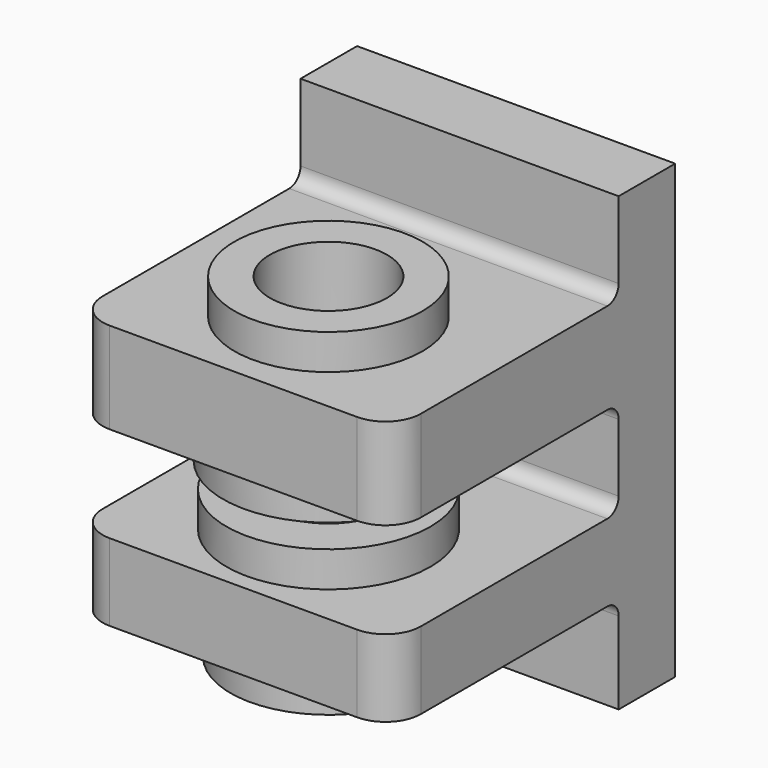
from build123d import *

# Parameters (mm, degrees)
F0_W       = 114.3609508872
F0_H       = 162.4245643616
F1_DEPTH   = 25.4
F2_W       = 114.3609508872
F2_H       = 32.8328199685
F2_H_2     = 27.7516581118
F3_DEPTH   = 101.6
F4_R       = 21.0436715378
F3_FACE1_W = 114.3609508872
F3_FACE1_H = 101.6
F5_DEPTH   = 228.6
F6_R       = 33.8173420759
F6_R_2     = 21.0436715378
F10_DEPTH  = 12.7
F9_R       = 35.2124743409
F9_R_2     = 21.0436715378
F11_DEPTH  = 12.7
F12_R      = 5.08
F7_R       = 37.8739843542
F7_R_2     = 21.0436715378
F13_DEPTH  = 12.7
F8_R       = 36.6649491414
F8_R_2     = 21.0436715378
F14_DEPTH  = 12.7
F15_R      = 12.7


with BuildPart() as f1:
    # F0 (on Front) → F1 (new body)
    with BuildSketch(Plane.XZ):
        Rectangle(F0_W, F0_H)
    extrude(amount=F1_DEPTH)

    # F2 (on face) → F3 (join)
    with BuildSketch(Plane.XZ.offset(25.4)):
        with Locations((0, 32.0948231965)):
            Rectangle(F2_W, F2_H)
        with Locations((0, -32.6631646603)):
            Rectangle(F2_W, F2_H_2)
    extrude(amount=F3_DEPTH)

    # F4 (on face) + F3_face1 (on face) → F5 (cut)
    with BuildSketch(Plane.XY.offset(48.5112331808)):
        with Locations((0, -84.3189582229)):
            Circle(F4_R)
    with BuildSketch(Plane(origin=(0, -76.2, -46.5389937162), x_dir=(1, 0, 0), z_dir=(0, 0, -1))):
        Rectangle(F3_FACE1_W, F3_FACE1_H)
    extrude(amount=-F5_DEPTH, dir=(0, 0, 1), mode=Mode.SUBTRACT)

    # F6 (on face) → F10 (join)
    with BuildSketch(Plane.XY.offset(48.5112331808)):
        with Locations((0, -84.3189582229)):
            Circle(F6_R)
        with Locations((0, -84.3189582229)):
            Circle(F6_R_2, mode=Mode.SUBTRACT)
    extrude(amount=F10_DEPTH)

    # F9 (on face) → F11 (join)
    with BuildSketch(Plane(origin=(0, 0, -46.5389937162), x_dir=(1, 0, 0), z_dir=(0, 0, -1))):
        with Locations((0, 84.3189582229)):
            Circle(F9_R)
        with Locations((0, 84.3189582229)):
            Circle(F9_R_2, mode=Mode.SUBTRACT)
    extrude(amount=F11_DEPTH)

    # F12
    f12_edges = [f1.edges().sort_by_distance(p)[0] for p in [
        (0, -25.4, 48.511233),
        (0, -25.4, 15.678413),
        (0, -25.4, -18.787336),
        (0, -25.4, -46.538994),
    ]]
    fillet(f12_edges, radius=F12_R)

    # F7 (on face) → F13 (join)
    with BuildSketch(Plane(origin=(0, 0, 15.6784132123), x_dir=(1, 0, 0), z_dir=(0, 0, -1))):
        with Locations((0, 84.3189582229)):
            Circle(F7_R)
        with Locations((0, 84.3189582229)):
            Circle(F7_R_2, mode=Mode.SUBTRACT)
    extrude(amount=F13_DEPTH)

    # F8 (on face) → F14 (join)
    with BuildSketch(Plane.XY.offset(-18.7873356044)):
        with Locations((0, -84.3189582229)):
            Circle(F8_R)
        with Locations((0, -84.3189582229)):
            Circle(F8_R_2, mode=Mode.SUBTRACT)
    extrude(amount=F14_DEPTH)

    # F15
    f15_edges = [f1.edges().sort_by_distance(p)[0] for p in [
        (57.180475, -127, -32.663165),
        (57.180475, -127, 32.094823),
        (-57.180475, -127, -32.663165),
        (-57.180475, -127, 32.094823),
    ]]
    fillet(f15_edges, radius=F15_R)


solid = f1.part
